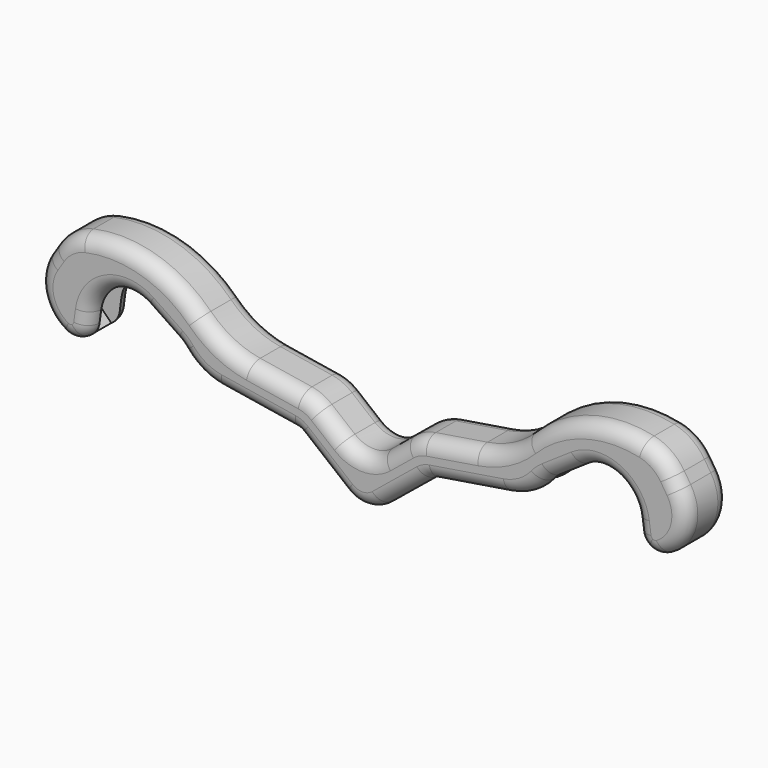
from build123d import *

# Parameters (mm, degrees)
F1_DEPTH = 4.5
F2_START = 2.1
F2_DEPTH = 2.4
F4_R     = 2.39999


# Not quite as in the source:
# - a fillet or chamfer is up to 0.001 mm smaller than in the source, because OpenCascade refuses the exact size


with BuildPart() as f1:
    # F0 (on Front) → F1 (new body, symmetric)
    with BuildSketch(Plane.XZ):
        with BuildLine():
            Line((-47.1743682614, 8.7650161883), (-50.090854948, 11.7506831815))
            ThreePointArc((-50.090854948, 11.7506831815), (-51.488428864, 14.7382643158), (-50.7214142363, 17.9461518522))
            Line((-50.7214142363, 17.9461518522), (-49.6606151776, 19.5981587494))
            ThreePointArc((-49.6606151776, 19.5981587494), (-46.2125472816, 21.9983199589), (-42.07601531, 21.2641201938))
            Line((-42.07601531, 21.2641201938), (-30.8393361164, 14.1006776114))
            ThreePointArc((-30.8393361164, 14.1006776114), (-29.2013263581, 13.2778210914), (-27.4305677415, 12.8039194748))
            Line((-27.4305677415, 12.8039194748), (-11.064559227, 10.1714510051))
            ThreePointArc((-11.064559227, 10.1714510051), (-9.8110357286, 9.7964249769), (-8.6977267313, 9.1090322513))
            Line((-8.6977267313, 9.1090322513), (-3.1608748809, 4.5915525411))
            ThreePointArc((-3.1608748809, 4.5915525411), (0, 3.4656808285), (3.1608748809, 4.5915525411))
            Line((3.1608748809, 4.5915525411), (8.6977267313, 9.1090322513))
            ThreePointArc((8.6977267313, 9.1090322513), (9.8110357286, 9.7964249769), (11.064559227, 10.1714510051))
            Line((11.064559227, 10.1714510051), (27.4305677415, 12.8039194748))
            ThreePointArc((27.4305677415, 12.8039194748), (29.2013263581, 13.2778210914), (30.8393361164, 14.1006776114))
            Line((30.8393361164, 14.1006776114), (42.07601531, 21.2641201938))
            ThreePointArc((42.07601531, 21.2641201938), (46.2125472816, 21.9983199589), (49.6606151776, 19.5981587494))
            Line((49.6606151776, 19.5981587494), (50.7214142363, 17.9461518522))
            ThreePointArc((50.7214142363, 17.9461518522), (51.488428864, 14.7382643158), (50.090854948, 11.7506831815))
            Line((50.090854948, 11.7506831815), (47.1743682614, 8.7650161883))
            ThreePointArc((47.1743682614, 8.7650161883), (48.6861089408, 8.3293539672), (50.2104483206, 8.718649366))
            ThreePointArc((50.2104483206, 8.718649366), (53.7950221227, 13.4449386002), (52.825058334, 19.2969595773))
            Line((52.825058334, 19.2969595773), (51.7642592753, 20.9489664745))
            ThreePointArc((51.7642592753, 20.9489664745), (49.6030454927, 23.1922793472), (46.7488877902, 24.440110052))
            ThreePointArc((46.7488877902, 24.440110052), (36.2348884349, 24.0758353702), (27.1917513421, 18.7000982107))
            ThreePointArc((27.1917513421, 18.7000982107), (23.4040745539, 15.9369537144), (18.9483734619, 14.4781217369))
            Line((18.9483734619, 14.4781217369), (10.3229105408, 13.0907181341))
            ThreePointArc((10.3229105408, 13.0907181341), (8.567977643, 12.5656816946), (7.0093450467, 11.6033318787))
            Line((7.0093450467, 11.6033318787), (3.1608748809, 8.4633912845))
            ThreePointArc((3.1608748809, 8.4633912845), (0, 7.3375195719), (-3.1608748809, 8.4633912845))
            Line((-3.1608748809, 8.4633912845), (-7.0093450467, 11.6033318787))
            ThreePointArc((-7.0093450467, 11.6033318787), (-8.567977643, 12.5656816946), (-10.3229105408, 13.0907181341))
            Line((-10.3229105408, 13.0907181341), (-18.9483734619, 14.4781217369))
            ThreePointArc((-18.9483734619, 14.4781217369), (-23.4040745539, 15.9369537144), (-27.1917513421, 18.7000982107))
            ThreePointArc((-27.1917513421, 18.7000982107), (-36.2348884349, 24.0758353702), (-46.7488877902, 24.440110052))
            ThreePointArc((-46.7488877902, 24.440110052), (-49.6030454927, 23.1922793472), (-51.7642592753, 20.9489664745))
            Line((-51.7642592753, 20.9489664745), (-52.825058334, 19.2969595773))
            ThreePointArc((-52.825058334, 19.2969595773), (-53.7950221227, 13.4449386002), (-50.2104483206, 8.718649366))
            ThreePointArc((-50.2104483206, 8.718649366), (-48.6861089408, 8.3293539672), (-47.1743682614, 8.7650161883))
        make_face()
    extrude(amount=F1_DEPTH, both=True)

    # F0 (on Front) → F2 (join)
    with BuildSketch(Plane.XZ.offset(F2_START)):
        with BuildLine():
            ThreePointArc((-50.7214142363, 17.9461518522), (-51.488428864, 14.7382643158), (-50.090854948, 11.7506831815))
            Line((-50.090854948, 11.7506831815), (-47.1743682614, 8.7650161883))
            ThreePointArc((-47.1743682614, 8.7650161883), (-46.2210159505, 9.6872478577), (-45.7585151015, 10.9304231653))
            Line((-45.7585151015, 10.9304231653), (-45.480066099, 13.0076456929))
            ThreePointArc((-45.480066099, 13.0076456929), (-41.988471743, 17.6851455651), (-36.1732737838, 17.1814503225))
            Line((-36.1732737838, 17.1814503225), (-31.3098625957, 13.8941656875))
            ThreePointArc((-31.3098625957, 13.8941656875), (-30.6277054349, 13.3572826148), (-30.0301617156, 12.7275816309))
            ThreePointArc((-30.0301617156, 12.7275816309), (-27.2812602678, 10.3986934149), (-23.8854388512, 9.1951252203))
            Line((-23.8854388512, 9.1951252203), (-11.5409846581, 7.2095227804))
            ThreePointArc((-11.5409846581, 7.2095227804), (-11.0395752587, 7.0595123691), (-10.5942516598, 6.7845552788))
            Line((-10.5942516598, 6.7845552788), (-3.1608748809, 0.7197137977))
            ThreePointArc((-3.1608748809, 0.7197137977), (0, -0.4061579148), (3.1608748809, 0.7197137977))
            Line((3.1608748809, 0.7197137977), (10.5942516598, 6.7845552788))
            ThreePointArc((10.5942516598, 6.7845552788), (11.0395752587, 7.0595123691), (11.5409846581, 7.2095227804))
            Line((11.5409846581, 7.2095227804), (23.8854388512, 9.1951252203))
            ThreePointArc((23.8854388512, 9.1951252203), (27.2812602678, 10.3986934149), (30.0301617156, 12.7275816309))
            ThreePointArc((30.0301617156, 12.7275816309), (30.6277054349, 13.3572826148), (31.3098625957, 13.8941656875))
            Line((31.3098625957, 13.8941656875), (36.1732737838, 17.1814503225))
            ThreePointArc((36.1732737838, 17.1814503225), (41.988471743, 17.6851455651), (45.480066099, 13.0076456929))
            Line((45.480066099, 13.0076456929), (45.7585151015, 10.9304231653))
            ThreePointArc((45.7585151015, 10.9304231653), (46.2210159505, 9.6872478577), (47.1743682614, 8.7650161883))
            Line((47.1743682614, 8.7650161883), (50.090854948, 11.7506831815))
            ThreePointArc((50.090854948, 11.7506831815), (51.488428864, 14.7382643158), (50.7214142363, 17.9461518522))
            Line((50.7214142363, 17.9461518522), (49.6606151776, 19.5981587494))
            ThreePointArc((49.6606151776, 19.5981587494), (46.2125472816, 21.9983199589), (42.07601531, 21.2641201938))
            Line((42.07601531, 21.2641201938), (30.8393361164, 14.1006776114))
            ThreePointArc((30.8393361164, 14.1006776114), (29.2013263581, 13.2778210914), (27.4305677415, 12.8039194748))
            Line((27.4305677415, 12.8039194748), (11.064559227, 10.1714510051))
            ThreePointArc((11.064559227, 10.1714510051), (9.8110357286, 9.7964249769), (8.6977267313, 9.1090322513))
            Line((8.6977267313, 9.1090322513), (3.1608748809, 4.5915525411))
            ThreePointArc((3.1608748809, 4.5915525411), (0, 3.4656808285), (-3.1608748809, 4.5915525411))
            Line((-3.1608748809, 4.5915525411), (-8.6977267313, 9.1090322513))
            ThreePointArc((-8.6977267313, 9.1090322513), (-9.8110357286, 9.7964249769), (-11.064559227, 10.1714510051))
            Line((-11.064559227, 10.1714510051), (-27.4305677415, 12.8039194748))
            ThreePointArc((-27.4305677415, 12.8039194748), (-29.2013263581, 13.2778210914), (-30.8393361164, 14.1006776114))
            Line((-30.8393361164, 14.1006776114), (-42.07601531, 21.2641201938))
            ThreePointArc((-42.07601531, 21.2641201938), (-46.2125472816, 21.9983199589), (-49.6606151776, 19.5981587494))
            Line((-49.6606151776, 19.5981587494), (-50.7214142363, 17.9461518522))
        make_face()
    extrude(amount=F2_DEPTH)

    # F3: F1 across plane


with BuildPart() as f1_1:
    add(f1.part)
    add(f1.part.mirror(Plane.XZ))

    # F4 (radius 2.4 in the source; OpenCascade refuses exactly that, so slightly less here)
    f4_edges = [f1_1.edges().sort_by_distance(p)[0] for p in [
        (0, -4.5, 7.33752),
        (0, 4.5, 7.33752),
        (-47.397135, 4.5, 8.642305),
        (-47.397135, -4.5, 8.642305),
        (47.397135, -4.5, 8.642305),
        (53.795022, -4.5, 13.444939),
        (52.294659, -4.5, 20.122963),
        (49.603045, -4.5, 23.192279),
        (36.234888, -4.5, 24.075835),
        (23.404075, -4.5, 15.936954),
        (14.635642, -4.5, 13.78442),
        (8.567978, -4.5, 12.565682),
        (5.08511, -4.5, 10.033362),
        (-5.08511, -4.5, 10.033362),
        (-8.567978, -4.5, 12.565682),
        (-14.635642, -4.5, 13.78442),
        (-23.404075, -4.5, 15.936954),
        (-36.234888, -4.5, 24.075835),
        (-49.603045, -4.5, 23.192279),
        (-52.294659, -4.5, 20.122963),
        (-53.795022, -4.5, 13.444939),
        (-45.619291, -4.5, 11.969034),
        (-41.988472, -4.5, 17.685146),
        (-33.741568, -4.5, 15.537808),
        (-30.627705, -4.5, 13.357283),
        (-27.28126, -4.5, 10.398693),
        (-17.713212, -4.5, 8.202324),
        (-11.039575, -4.5, 7.059512),
        (-6.877563, -4.5, 3.752135),
        (0, -4.5, -0.406158),
        (6.877563, -4.5, 3.752135),
        (11.039575, -4.5, 7.059512),
        (17.713212, -4.5, 8.202324),
        (27.28126, -4.5, 10.398693),
        (30.627705, -4.5, 13.357283),
        (33.741568, -4.5, 15.537808),
        (41.988472, -4.5, 17.685146),
        (45.619291, -4.5, 11.969034),
        (-52.294659, 4.5, 20.122963),
        (-49.603045, 4.5, 23.192279),
        (-36.234888, 4.5, 24.075835),
        (-23.404075, 4.5, 15.936954),
        (-14.635642, 4.5, 13.78442),
        (-8.567978, 4.5, 12.565682),
        (-5.08511, 4.5, 10.033362),
        (5.08511, 4.5, 10.033362),
        (8.567978, 4.5, 12.565682),
        (14.635642, 4.5, 13.78442),
        (23.404075, 4.5, 15.936954),
        (36.234888, 4.5, 24.075835),
        (49.603045, 4.5, 23.192279),
        (52.294659, 4.5, 20.122963),
        (53.795022, 4.5, 13.444939),
        (47.397135, 4.5, 8.642305),
        (45.619291, 4.5, 11.969034),
        (41.988472, 4.5, 17.685146),
        (33.741568, 4.5, 15.537808),
        (30.627705, 4.5, 13.357283),
        (27.28126, 4.5, 10.398693),
        (17.713212, 4.5, 8.202324),
        (11.039575, 4.5, 7.059512),
        (6.877563, 4.5, 3.752135),
        (0, 4.5, -0.406158),
        (-6.877563, 4.5, 3.752135),
        (-11.039575, 4.5, 7.059512),
        (-17.713212, 4.5, 8.202324),
        (-27.28126, 4.5, 10.398693),
        (-30.627705, 4.5, 13.357283),
        (-33.741568, 4.5, 15.537808),
        (-41.988472, 4.5, 17.685146),
        (-45.619291, 4.5, 11.969034),
        (-53.795022, 4.5, 13.444939),
    ]]
    fillet(f4_edges, radius=F4_R)


solid = f1_1.part
